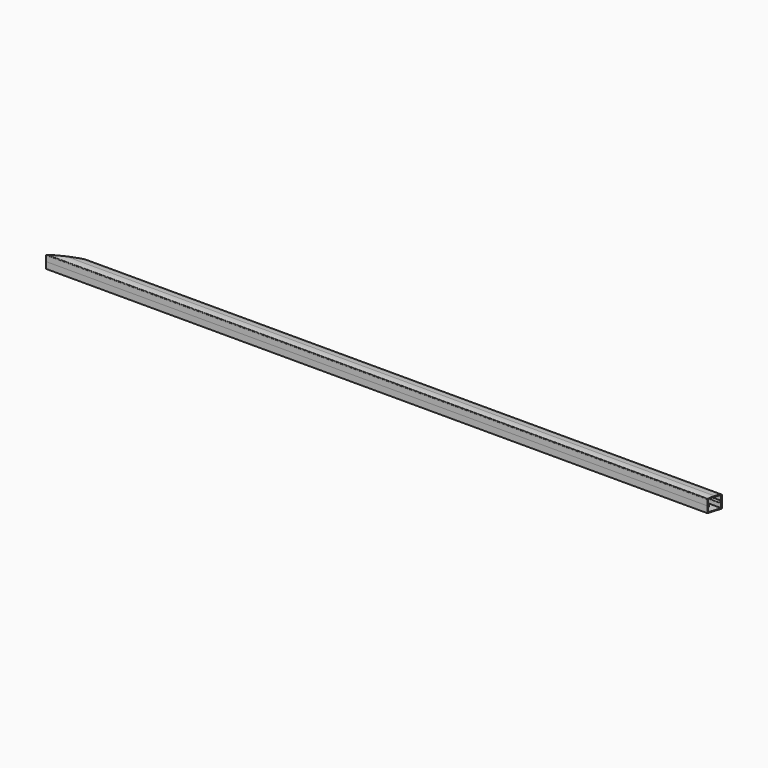
from build123d import *

# Parameters (mm, degrees)
F2_DEPTH      = 1200
F4_DEPTH      = 1200
F8_DEPTH      = 10.001
F8_DEPTH_BACK = 10.001


with BuildPart() as f2:
    # F1 (on Right) → F2 (new body)
    with BuildSketch(Plane.YZ):
        with BuildLine():
            Line((0, -9), (0, -10))
            Line((0, -10), (10, -10))
            Line((10, -10), (10, -0.2))
            Line((10, -0.2), (9, -0.2))
            ThreePointArc((9, -0.2), (8.5, -0.7), (9, -1.2))
            ThreePointArc((9, -1.2), (9.5, -1.7), (9, -2.2))
            Line((9, -2.2), (9, -9))
            Line((9, -9), (0, -9))
        make_face()
    extrude(amount=F2_DEPTH)

    # F5: F2 across plane


with BuildPart() as f4:
    # F3 (on Right) → F4 (new body)
    with BuildSketch(Plane.YZ):
        with BuildLine():
            Line((9, -0.2), (10, -0.2))
            Line((10, -0.2), (10, 8.1663783152))
            ThreePointArc((10, 8.1663783152), (9.7693092582, 8.8052548802), (9.1836734694, 9.1493656277))
            ThreePointArc((9.1836734694, 9.1493656277), (4.6114920912, 9.7868872364), (0, 10))
            Line((0, 10), (0, 9))
            ThreePointArc((0, 9), (4.5192622493, 8.7911494917), (9, 8.1663783152))
            Line((9, 8.1663783152), (9, 0.8))
            ThreePointArc((9, 0.8), (7.5, -0.7), (9, -2.2))
            ThreePointArc((9, -2.2), (9.5, -1.7), (9, -1.2))
            ThreePointArc((9, -1.2), (8.5, -0.7), (9, -0.2))
        make_face()
    extrude(amount=F4_DEPTH)

    # F6: F4 across plane


with BuildPart() as f2_1:
    add(f2.part)
    add(f2.part.mirror(Plane.XZ))


with BuildPart() as f4_1:
    add(f4.part)
    add(f4.part.mirror(Plane.XZ))


with BuildPart() as f8_tool:
    # F7 (on Top) → F8 (new body, two sides)
    with BuildSketch(Plane.XY) as f8_sk:
        Polygon((0, 10), (0, 0), (0, -10), (44.5020182264, 10), align=None)
        Polygon((1010.4383560074, 10), (1004.4, -10), (1208.0904245377, -10), (1208.0904245377, 10), align=None)
    extrude(amount=F8_DEPTH)
    extrude(f8_sk.sketch, amount=-F8_DEPTH_BACK)


with BuildPart() as f2_2:
    add(f2_1.part)

    # F8: cut by f8_tool
    add(f8_tool.part, mode=Mode.SUBTRACT)


with BuildPart() as f4_2:
    add(f4_1.part)

    # F8: cut by f8_tool
    add(f8_tool.part, mode=Mode.SUBTRACT)


solid = Compound([f2_2.part, f4_2.part])
